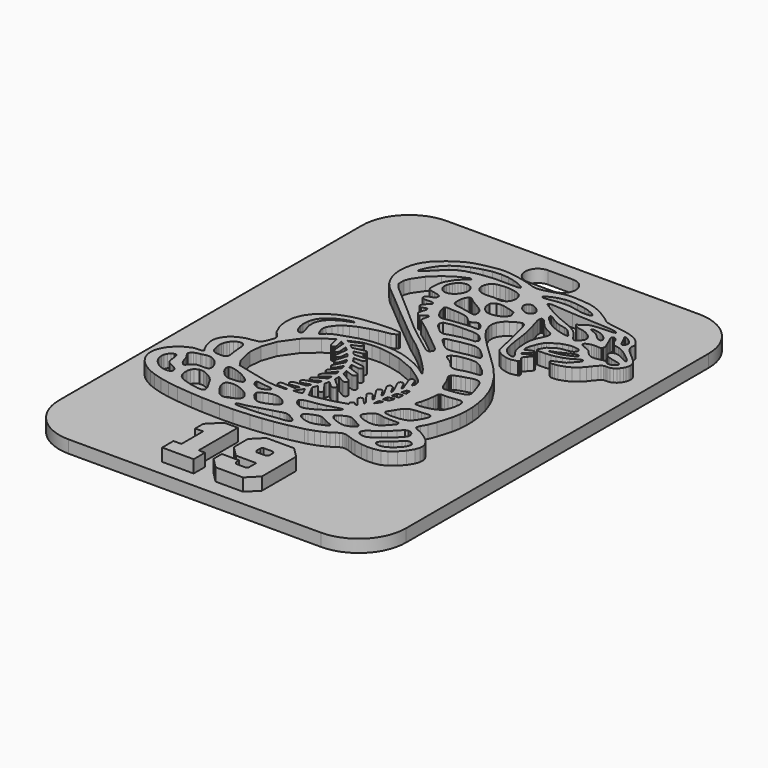
from build123d import *

# Parameters (mm, degrees)
F1_DEPTH = 2.54
F2_W     = 69.85
F2_H     = 95.25
F3_DEPTH = 2.54
F4_R     = 9.525
F6_DEPTH = 2.54


# Not quite as in the source:
# - ends of sketch curves that miss each other by under 0.0002 mm in the source are joined


with BuildPart() as f1:
    # F0 (on Top) → F1 (new body)
    with BuildSketch(Plane.XY):
        Polygon((-8.2281780429, 31.2462601157), (-10.0958576986, 30.7675389293), (-11.1380639944, 30.3636480727), (-12.4204415795, 29.652883082), (-13.8704177588, 28.6461216518), (-15.2257169463, 27.4888991275), (-15.8284643763, 26.846827805), (-16.5017936781, 25.9114281568), (-16.9868772898, 24.9886917871), (-17.2888461994, 24.1974729035), (-17.5726924591, 23.0136513372), (-17.6335459776, 22.5497689682), (-17.6740602593, 21.6151492301), (-17.6280045105, 20.8667022631), (-17.4269723981, 19.7555765356), (-17.20430804, 19.0304242543), (-16.7360745931, 17.9797210423), (-16.2140889153, 17.1404145386), (-15.6879573991, 16.5027353419), (-14.947678965, 15.7886249469), (-14.0724965927, 15.0634110938), (-12.5609690806, 13.8050465328), (-9.0886857893, 10.8515677067), (-5.342140924, 7.7478125022), (-2.8091978797, 5.6307257787), (-1.5091902196, 4.6283359503), (0.1423311709, 3.4050673477), (1.563163338, 2.2145549728), (3.5199169465, 0.3846804372), (5.5455078909, -1.6626453726), (6.1076589433, -2.2972254525), (6.8524115989, -3.2890454455), (7.0789960319, -3.6056479331), (7.0395079477, -3.7197611077), (6.1721041534, -3.0787570307), (5.0096069734, -2.3217515755), (3.8088120985, -1.7146325437), (1.7273139082, -0.8504920577), (0.0306808706, -0.3511648232), (-1.4594196354, -0.0862826953), (-2.7848359484, 0.0338439973), (-4.4325809316, 0.0443522608), (-6.0681552112, -0.0942459888), (-7.6592130383, -0.3793647336), (-9.5361079486, -0.9377804267), (-11.8733961559, -1.7510830829), (-12.6301963716, -2.0678087142), (-13.172562334, -2.4256438218), (-13.62142117, -2.8594996487), (-13.8745841211, -3.0896347254), (-14.0119304096, -3.1911872411), (-14.185008899, -3.1720383937), (-14.4263295297, -2.6863595874), (-14.7089238284, -1.8951612278), (-14.7727943678, -1.2952461032), (-14.6445196662, -0.7206575357), (-14.147203779, 0.1498248515), (-13.4946241929, 0.8740946028), (-12.8925335294, 1.3693170469), (-12.0459410226, 1.8987118715), (-10.7370054432, 2.4979291817), (-8.958543408, 3.0819382433), (-7.4131513747, 3.4864653423), (-6.2016635207, 3.7161283681), (-5.2402600249, 3.9098744774), (-4.4449568748, 4.2413363065), (-4.2034515286, 4.5321812339), (-4.2377060049, 4.9084058028), (-4.4755170398, 5.1506500113), (-5.1994789318, 5.2198157305), (-6.0173789533, 5.3073709108), (-7.4621420487, 5.2495344133), (-9.2230561048, 5.1676848917), (-12.0609850796, 4.8602976587), (-13.9591838523, 4.4160977599), (-15.9473596317, 3.6696210923), (-17.7325124754, 2.6187536887), (-19.0329100906, 1.4390779606), (-19.8561873876, 0.3138112301), (-20.3619796671, -0.7178252303), (-20.6945703135, -1.8480587573), (-20.7833158831, -3.0535330933), (-20.6529682622, -4.2906348398), (-20.3346828106, -5.4881458823), (-19.720175156, -6.8209097702), (-18.8984371554, -7.7585670532), (-18.5574522125, -8.2426244673), (-18.5128126164, -8.5026424185), (-18.66171389, -9.0847427525), (-19.0896998665, -10.1552105305), (-19.3077873832, -10.6363124954), (-19.3952194198, -10.823080461), (-19.5230836424, -10.9713249682), (-20.0220619698, -11.1893303891), (-21.0657459901, -11.3813114385), (-22.2214497419, -11.5752627874), (-23.3337863825, -11.996332192), (-24.0131702503, -12.3898584526), (-24.7578613341, -13.0130887869), (-25.3504699316, -13.7868007393), (-25.6892382876, -14.5173918679), (-25.8122793814, -15.0092073359), (-25.8467801452, -15.595576652), (-25.7631450397, -16.2746937083), (-25.5535954872, -17.0447113492), (-25.4211133753, -17.4274420109), (-25.0605075341, -18.2154181101), (-24.7159924715, -18.7689080546), (-24.6677201357, -18.8595213039), (-24.6881209443, -19.0501888204), (-25.0308504231, -19.1392012013), (-25.7215840364, -19.1855032376), (-26.1809716599, -19.2103782678), (-26.5443892825, -19.2721143162), (-27.3716892742, -19.6063468787), (-28.0206771686, -19.9679994415), (-28.7905100939, -20.5251016016), (-29.4208211918, -21.1146316064), (-29.9690570046, -21.7761596356), (-30.3697256006, -22.415706512), (-30.7029935374, -23.1830765631), (-30.8776934191, -23.8991367335), (-30.9240570272, -24.5455386099), (-30.876441458, -25.1101935845), (-30.7473663222, -25.6701896219), (-30.4887029519, -26.3609437592), (-30.2370587732, -26.8394802301), (-29.6598020919, -27.6332235598), (-29.088415261, -28.206642262), (-28.1307676485, -28.9230923875), (-26.9608202739, -29.5598274824), (-25.6898745302, -30.0719206153), (-24.0739621969, -30.5487535982), (-22.1714328702, -30.9419104277), (-20.1395410725, -31.2260645467), (-17.1374204796, -31.5122300131), (-14.8925105813, -31.6548509573), (-11.3057036364, -31.75), (-8.6367688845, -31.7091162871), (-5.3569386935, -31.5193518245), (-3.1109205019, -31.2946966431), (-0.9777019518, -31.0051652485), (1.5435424396, -30.5608011581), (4.337406489, -29.9279040423), (4.9370958501, -29.7589919152), (5.9386031485, -29.4248824963), (6.9207768839, -29.0279903075), (7.7674309626, -28.6199536126), (8.2726280474, -28.3307916492), (8.9759223196, -27.8459132771), (9.5296995994, -27.5060776756), (9.9716829114, -27.331767749), (10.2292790362, -27.2936137218), (10.7020482765, -27.3414755784), (11.3129642395, -27.5130147714), (12.2242277198, -27.8546359568), (13.03843343, -28.0966133539), (14.6348685326, -28.3984591198), (15.7869805927, -28.5070923992), (16.9305136408, -28.4916173392), (18.3728343859, -28.2090640884), (19.3723098131, -27.7017530364), (20.5650798226, -26.7484154539), (21.4969288271, -25.7102113288), (22.2529696565, -24.485731813), (22.5528861709, -23.6063009826), (22.6021436563, -22.830167204), (22.4525445683, -22.2410271543), (22.1046430535, -21.6120501134), (21.5689678995, -20.9829088808), (20.7981293005, -20.3279895641), (19.6320814768, -19.5857203067), (18.0839597578, -18.8412960343), (17.8310430941, -18.6388682931), (17.7820318961, -18.4662208067), (17.8314125253, -18.1861304302), (17.9895906253, -17.781664903), (18.6505850318, -16.6351148339), (19.2241063538, -15.1447475166), (20.0612988904, -12.3389180031), (20.3419228897, -10.7201733644), (20.434650106, -9.2487907029), (20.4032279351, -7.6929725018), (20.2038172149, -5.9142436552), (19.6753254442, -3.6030824391), (19.0529776398, -1.8339793261), (18.1165928419, 0.1336314532), (16.4870115564, 2.6515509644), (14.4028042044, 5.0404158638), (11.7791042432, 7.596161019), (8.9855275292, 10.2726691093), (6.7964222572, 12.5526954898), (5.7074418742, 14.12870926), (5.1848404778, 15.5236607232), (5.1331816899, 16.344885625), (5.352849551, 17.23264918), (6.032541278, 18.1864793374), (6.7197037236, 18.7081571559), (7.7446698995, 19.31689758), (8.4808435431, 19.6174913848), (8.7462798177, 19.662110457), (9.053954386, 19.5342051865), (9.2906776514, 19.1477391655), (9.5775204082, 18.2618022422), (9.8677290932, 16.9917595524), (10.834263577, 13.1887532943), (11.0390926205, 11.8791609485), (11.4717170102, 10.3329069092), (11.9607001728, 9.7361524732), (12.7906067064, 9.2087895199), (13.9503742007, 8.8610727207), (14.9139942833, 8.7772939476), (16.1735287096, 9.0840038902), (16.347448681, 9.2895102242), (16.3674595345, 9.5117435792), (16.221924189, 9.7619100333), (15.9084618661, 10.1001858145), (15.837572135, 10.2823769387), (15.8998828541, 10.5336722102), (16.0684871219, 10.7846596224), (16.4075633372, 11.1428231133), (17.0936174894, 11.9521441227), (17.0494499441, 12.3008460717), (16.732683265, 12.2797679727), (15.8150984073, 11.7842787172), (15.0990177129, 11.3454971418), (14.8941476215, 11.4280650018), (14.9146510498, 11.670863357), (15.3561417869, 12.0663599171), (15.8215429283, 12.3852200394), (16.3334308216, 12.9318344599), (16.3681368249, 13.2268252258), (15.9950524207, 13.3743308707), (15.3028205589, 13.0950204044), (14.6702313023, 12.792948875), (14.4427848634, 12.7538507459), (14.3894841594, 12.9031214507), (14.3610584855, 13.1483416323), (14.353936674, 13.4823894793), (14.4100491595, 13.7212472357), (14.498835777, 14.1628200686), (14.7819842224, 14.9135246704), (15.0271017842, 15.5714199601), (15.3040314721, 16.0905733326), (15.5397285398, 16.4512612696), (15.7826705627, 16.6768605528), (16.1297305955, 16.8937576803), (17.1537116216, 17.6541085397), (17.995316808, 18.0185113121), (18.999615364, 18.2874777065), (19.7587758341, 18.3525386351), (20.4528958996, 18.2983143533), (21.0168530598, 18.2007024363), (21.3530559218, 17.9078872094), (21.3694956075, 17.615277222), (21.2827203374, 17.2942620847), (20.9964112033, 17.0079324267), (20.484502786, 16.8344024104), (19.7045515523, 16.7040342656), (19.0104520108, 16.6281161662), (18.424801033, 16.4546066738), (17.7849257734, 16.205158558), (16.754602846, 15.4025899288), (16.2994021088, 14.6136697279), (16.0761630801, 14.2962257583), (16.0630893225, 14.0488916096), (16.136790835, 13.9380827914), (16.269231899, 13.8613232099), (16.4453479333, 13.8129893023), (16.8682029217, 13.7790426853), (17.8758674059, 13.8107111436), (18.9218295849, 13.9036846474), (19.8006446967, 14.0631352325), (20.9053669511, 14.3650220463), (21.9472448636, 14.7667784118), (22.7663147504, 15.2334930862), (23.4398082439, 15.6252748109), (23.7038899376, 15.6872776707), (23.9646467511, 15.7318967429), (24.1143484589, 15.5621841816), (24.1351802704, 15.2637248679), (23.8644693401, 14.9652450301), (23.5979863439, 14.656195357), (23.1121022981, 14.0939622088), (22.4531397629, 13.4007246733), (21.5882809386, 13.0305751943), (20.6687257815, 12.6129948616), (20.2689191915, 12.4486390519), (20.1267702982, 12.3242433772), (20.124266376, 12.1040829413), (20.3203522159, 11.9487781946), (20.6240246135, 11.786084825), (20.9493908287, 11.7535543607), (21.3615117901, 11.786084825), (22.0122442205, 11.883696742), (23.1888413556, 12.2794395894), (24.0884061832, 12.7236600122), (25.0990261164, 13.4955042848), (25.8153325743, 14.2562450993), (26.2896821589, 14.8887522601), (26.9574084218, 15.6792117574), (27.3181374067, 16.0484376586), (27.6401171698, 16.2497571063), (27.9280887439, 16.3047612984), (28.3638532983, 16.2896351455), (28.8693582425, 16.3261883045), (29.4282049386, 16.5455688302), (29.9020209005, 16.884029327), (30.2338316366, 17.2422338657), (30.5140656808, 17.6528976265), (30.7363606077, 18.0986573457), (30.8880941868, 18.590760149), (30.9240316272, 18.9710895083), (30.867364995, 19.395114362), (30.6497700532, 19.9153555039), (30.1435057228, 20.5675861828), (29.0852291724, 21.5027395436), (28.2911985073, 22.1658889651), (27.6971532331, 22.7558499728), (27.3140120923, 23.2695439739), (27.0744359976, 23.7597790976), (27.0528447998, 24.0224241147), (27.1311231537, 24.3673291324), (27.1803806391, 24.6259514549), (27.1202044111, 24.8888017115), (26.8265271782, 25.3891346197), (26.2102749876, 26.0746551491), (25.6260606865, 26.5040778023), (24.7185941374, 26.9510689585), (23.6292237993, 27.28835959), (22.4830021134, 27.5173863733), (19.8549921223, 27.9070541309), (19.0187847354, 28.0869055245), (18.4877479946, 28.3549072931), (17.6594833772, 29.0080410259), (16.1305720775, 29.964990824), (14.8880930556, 30.6054202303), (13.9080538112, 30.9904290508), (12.8522401351, 31.2396514031), (11.0529668122, 31.4290464346), (9.4259304968, 31.5157396089), (8.1718759658, 31.4638550576), (6.8842647728, 31.1987061183), (5.5986033554, 30.7903820881), (3.8220910956, 30.3162993149), (3.052812317, 30.2314738202), (2.5093585851, 30.2679448833), (1.9189050025, 30.4165793456), (0.5883577014, 30.8681268193), (-0.7917549444, 31.2065462681), (-2.3376806005, 31.5184282466), (-3.3967370611, 31.6696487269), (-4.5497521751, 31.75), (-5.5576834706, 31.7197682183), align=None)
        Polygon((-26.759582922, -24.733825348), (-26.6166335945, -25.1517956357), (-26.3761133979, -25.4887784079), (-26.0296690838, -25.7474417782), (-25.2160585683, -26.1086017662), (-24.8611583858, -26.2953286838), (-24.5108760926, -26.5698775932), (-24.2769030368, -26.8857412185), (-24.1925085451, -27.1663241698), (-24.2551886953, -27.4858000107), (-24.5195372004, -27.7267922582), (-25.0954803488, -27.8368416902), (-25.7274949347, -27.7817964502), (-26.3844461226, -27.5969166883), (-27.0999726702, -27.2360645596), (-27.962450716, -26.4982284759), (-28.4078204801, -25.8707291595), (-28.6838060661, -25.1937465942), (-28.7662097345, -24.514998969), (-28.7052946442, -23.9864866743), (-28.4672988937, -23.4257722985), (-28.049739085, -22.9743684925), (-27.5664410572, -22.7001069185), (-27.2383451564, -22.6899065142), (-26.9941306484, -22.9745737321), (-26.8677441504, -23.5810154734), align=None, mode=Mode.SUBTRACT)
        Polygon((-22.202916613, -27.5599325263), (-22.3819265246, -26.9413611291), (-22.4322102076, -26.0260749541), (-22.2596858649, -25.3087628226), (-21.9461824942, -24.8590625046), (-21.2046315751, -24.4321642976), (-20.3707023468, -24.4497328008), (-19.4872898697, -24.7880906777), (-18.3880269866, -25.4511990513), (-17.6717410527, -26.1620871857), (-16.7023126917, -27.8573245945), (-16.3128706975, -28.6299282534), (-16.200461011, -29.1731356979), (-16.4079992162, -29.4533697421), (-16.8004582314, -29.536389129), (-17.5492335817, -29.513176539), (-18.9130912573, -29.2795934383), (-20.8303157337, -28.7326711584), (-21.7562743639, -28.1908798667), align=None, mode=Mode.SUBTRACT)
        Polygon((-24.342148681, -20.2197872878), (-24.0994734695, -20.1636748023), (-23.470722192, -19.970359696), (-22.7253332938, -19.9014402643), (-22.2301929456, -20.025835939), (-21.7044103365, -20.2916005968), (-21.1895259462, -20.6784770969), (-20.7276754485, -21.1654283882), (-20.293224427, -21.8756597562), (-20.1027621501, -22.4481754045), (-20.0719556977, -22.8336152279), (-20.1209668957, -23.0471259033), (-20.3133173763, -23.2723762794), (-20.6286268549, -23.3885828971), (-21.0614359601, -23.4046941996), (-22.050731507, -23.3767816245), (-22.5260251934, -23.4221806069), (-22.8593547021, -23.5455706079), (-23.1443092553, -23.7368948909), (-23.427293509, -24.0120389949), (-23.7964783623, -24.4547406451), (-23.9932825405, -24.6317802573), (-24.1245742631, -24.6750037008), (-24.2582262402, -24.6569631467), (-24.457390673, -24.5295299272), (-24.7080702259, -24.2376382781), (-24.8213624424, -24.0560628725), (-25.0115168601, -23.6667029741), (-25.1196575645, -23.3783824928), (-25.2839107545, -22.8382331172), (-25.4733057859, -22.3513228738), (-25.8051165221, -21.8535554596), (-26.0125521076, -21.527511954), (-26.0798501471, -21.2741027154), (-26.0156101765, -21.0225816805), (-25.8401714326, -20.7860020828), (-25.5214960258, -20.5403508982), (-25.0908008876, -20.3568872889), align=None, mode=Mode.SUBTRACT)
        Polygon((-17.1074965572, -23.2132262489), (-17.7370277449, -22.5083926804), (-17.9198961595, -22.2233765554), (-18.1460701134, -21.760951387), (-18.2215366859, -21.5082810107), (-18.2521584226, -21.2161020263), (-18.2186222847, -21.040847998), (-18.1265723588, -20.9170680419), (-17.9316769081, -20.8158233854), (-17.7361657389, -20.7829645378), (-17.4117025776, -20.7937806607), (-16.8161385309, -20.9027012753), (-15.9991005154, -21.1578140019), (-15.2389343715, -21.4770230314), (-14.3613301729, -21.9438813735), (-13.8178969649, -22.3136408974), (-13.5455030705, -22.5398353753), (-13.3366102844, -22.7629102124), (-13.1619104028, -23.0452787476), (-13.1210472139, -23.23857333), (-13.1484672141, -23.353774274), (-13.2810108978, -23.5005000087), (-13.5042088786, -23.6188616414), (-13.9271459628, -23.7302040824), (-14.6808265377, -23.8235675413), (-15.3930487291, -23.8550923319), (-15.9068863979, -23.8169793526), (-16.1946116846, -23.7538887233), (-16.4728138575, -23.6440855787), align=None, mode=Mode.SUBTRACT)
        Polygon((-12.8974592779, -25.1261201715), (-12.3701578965, -25.2927541399), (-11.5050938326, -25.6835301909), (-10.7132387065, -26.2278664527), (-10.1603644805, -26.8242104096), (-9.9091718288, -27.2781386618), (-9.8396572025, -27.5718364186), (-9.8663588644, -27.8504901184), (-10.0593250636, -28.1672978455), (-10.4926267437, -28.5056967704), (-11.726342038, -29.1017533919), (-12.2817407101, -29.2628458932), (-12.7144882435, -29.2847859982), (-13.0222449077, -29.2106329587), (-13.5003708995, -28.9325744535), (-13.9346372054, -28.5016535518), (-14.6941671067, -27.4812847412), (-15.0965391908, -26.7685494511), (-15.2954573361, -26.1941866471), (-15.3317231597, -25.8460593688), (-15.2452762728, -25.4747195006), (-15.0617510917, -25.2422652173), (-14.8546233655, -25.1114455456), (-14.4884760571, -25.0028122663), (-14.0466569368, -24.9644324756), (-13.4231392672, -25.0146751107), align=None, mode=Mode.SUBTRACT)
        Polygon((-4.851166938, -30.08710834), (-6.5055616818, -30.1622875771), (-7.2232637684, -30.1749919035), (-7.8778957497, -30.2128996434), (-8.6038484651, -30.2237157662), (-8.9476862373, -30.2029660505), (-9.198899413, -30.158449598), (-9.3357120787, -30.1119628462), (-9.4727710319, -30.0381792378), (-9.5219669455, -29.8129493857), (-9.3118427222, -29.698446256), (-8.8494380778, -29.6002186205), (-7.6896911074, -29.3679695767), (-5.8136992511, -28.818399707), (-3.5194087237, -28.1618179503), (-2.2662572466, -27.8017457318), (-1.61476543, -27.6151624818), (-1.275155592, -27.5744429605), (-1.0524091381, -27.5818521073), (-0.7409786865, -27.6384161197), (-0.3543074259, -27.7892671689), (0.4216621612, -28.2636167535), (0.8223307572, -28.5158766507), (1.0612295615, -28.7540981646), (1.111739008, -28.9923402024), (0.9787437974, -29.194583228), (0.6180763843, -29.3989196967), (0.0708257212, -29.5412122577), (-0.6144690447, -29.6229591596), (-1.163361624, -29.6759314804), (-3.0051400519, -29.9139682787), align=None, mode=Mode.SUBTRACT)
        Polygon((-5.9171604944, -26.9613719826), (-6.6794611293, -27.1745132268), (-7.1504242618, -27.204108766), (-7.5577426184, -27.1141112353), (-7.9953132806, -26.8809591376), (-8.4064080443, -26.5396252876), (-8.8387040508, -26.0707350742), (-9.1802841883, -25.560550669), (-9.2703843387, -25.2923231369), (-9.2655612099, -25.0973250664), (-9.1131092925, -24.8225914415), (-8.8577913264, -24.6013021882), (-8.4295385385, -24.3461484137), (-7.6373755531, -23.9981237552), (-6.8443095138, -23.7952239632), (-6.3217902132, -23.7631655498), (-5.8916697457, -23.8098985891), (-5.4507126314, -23.9300868535), (-4.9985494392, -24.1331508372), (-4.4363368149, -24.5087186396), (-4.0562126951, -24.8704738221), (-3.8509936964, -25.1563724771), (-3.763500088, -25.4378584823), (-3.7734747287, -25.6164989628), (-3.8925752237, -25.8666859409), (-4.1326438933, -26.0924494157), (-4.5617176393, -26.3645559748), (-5.3110266123, -26.7172806183), align=None, mode=Mode.SUBTRACT)
        Polygon((-10.5022730012, -22.082520671), (-9.9462791345, -22.1563248033), (-9.2089561496, -22.2253879027), (-8.7606514603, -22.2807820498), (-8.3507265618, -22.3887996106), (-8.2321391657, -22.4864730994), (-8.1978025936, -22.644404912), (-8.2847831032, -22.8226554374), (-8.4619663831, -23.0065090018), (-8.8382525238, -23.261354917), (-9.219936464, -23.4272294992), (-9.554415314, -23.509407404), (-9.9007570084, -23.5342413862), (-10.2455388824, -23.5004589608), (-10.6516668497, -23.381727897), (-11.0075727059, -23.1915734793), (-11.2879709417, -22.9428231779), (-11.4925742218, -22.6724611548), (-11.6259388635, -22.3687887571), (-11.6433226511, -22.2036530373), (-11.5733770218, -22.0553469582), (-11.4407922902, -21.9896292631), (-11.2334182766, -21.9775817031), (-10.9516038881, -22.0096811644), align=None, mode=Mode.SUBTRACT)
        with BuildLine():
            Line((-4.2176746275, -20.7893064391), (-5.2175194858, -20.8481486102))
            ThreePointArc((-5.2175194858, -20.8481486102), (-4.6245377337, -20.0558732964), (-4.0970094123, -19.2185906677))
            Line((-4.0970094123, -19.2185906677), (-3.4045772108, -20.5774376799))
            Line((-3.4045772108, -20.5774376799), (-4.2176746275, -20.7893064391))
        make_face(mode=Mode.SUBTRACT)
        Polygon((-21.4224933283, -18.4982586962), (-22.2189458197, -18.4766880224), (-22.8653066482, -18.3592089196), (-23.1687532824, -18.2381791731), (-23.316833598, -18.1247843369), (-23.489234797, -17.9098164609), (-23.7110166251, -17.4077390168), (-23.9041059679, -16.6321799088), (-23.9764528997, -15.9574755022), (-23.9532813576, -15.4659678934), (-23.8623602491, -15.0254007342), (-23.6257190795, -14.4605610441), (-23.3892010536, -14.0834949931), (-22.9616255562, -13.6342667261), (-22.3591038897, -13.2917014389), (-21.8191392297, -13.1782039829), (-21.4304771457, -13.2410278007), (-21.185749539, -13.4034748829), (-21.0409735797, -13.5936087766), (-20.9108517224, -13.9666931808), (-20.8636466322, -14.3503474204), (-20.8267035181, -15.0055745963), (-20.6767760469, -16.3550655053), (-20.5291062104, -17.3481579834), (-20.5083154467, -17.8523699185), (-20.6542407473, -18.2021801609), (-20.9341669322, -18.3922730067), align=None, mode=Mode.SUBTRACT)
        Polygon((-12.825194442, -4.1463719793), (-10.7946777491, -2.9304099037), (-10.2791571162, -4.9154249945), (-10.1506361272, -5.1399775562), (-9.9203573828, -5.2698531261), (-9.6619197759, -5.2637164643), (-9.3606486807, -5.0298665523), (-9.3128894438, -4.6639860553), (-9.7389256448, -3.0235270751), (-8.9664656536, -3.4575470936), (-8.8077744547, -5.873483086), (-8.7207939451, -6.1222333874), (-8.5300032848, -6.2849883288), (-8.2534635521, -6.3299357843), (-7.9269685195, -6.1580271601), (-7.8115007641, -5.8075806753), (-7.9182047919, -4.1829046144), (-7.2518741578, -4.7418744542), (-7.5419596991, -7.0903071676), (-7.5047292497, -7.3473286218), (-7.3546786347, -7.5401511533), (-7.0896528392, -7.6419499565), (-6.7300937195, -7.5348559736), (-6.5509811881, -7.212239968), (-6.3574608423, -5.6455440722), (-5.8134119158, -6.3070310535), (-6.5265782089, -8.5227558917), (-6.5361423707, -8.7908192321), (-6.4230964416, -9.0040220482), (-6.192058311, -9.1475870943), (-5.8123857181, -9.1115675581), (-5.57601136, -8.8282343971), (-5.101805443, -7.354984056), (-4.6920652601, -8.0958782086), (-5.7976084725, -10.1200940482), (-5.8576205089, -10.3721281819), (-5.778049146, -10.6250653696), (-5.5741847282, -10.8025154608), (-5.2063955037, -10.8322957156), (-4.9211125673, -10.5982816119), (-4.184774732, -9.2501042358), (-3.9177375892, -10.0471519218), (-5.3808490979, -11.8257576247), (-5.4845771526, -12.0477857403), (-5.4621034249, -12.3104718053), (-5.2998205344, -12.529831807), (-4.9335706063, -12.6361253558), (-4.6094768762, -12.4597014621), (-3.6285345779, -11.2672393119), (-3.5095982745, -12.0971868934), (-5.2910978547, -13.5792830579), (-5.437577302, -13.7857745416), (-5.4617339938, -14.040107358), (-5.3345675856, -14.2959999948), (-5.0035778075, -14.4591038434), (-4.6521666969, -14.3465299653), (-3.4445578698, -13.3418825022), (-3.4764315677, -14.1813737215), (-5.5314949075, -15.3185648683), (-5.7228397144, -15.5089860974), (-5.7849041461, -15.723687162), (-5.7153484719, -16.0030386762), (-5.413933709, -16.2366833487), (-5.0476632569, -16.1919616567), (-3.6343018085, -15.4098554079), (-3.8170676033, -16.2353492918), (-6.0935433402, -16.9819901511), (-6.3025797939, -17.1165657061), (-6.4267086572, -17.3739155435), (-6.3978109324, -17.6323941982), (-6.1501073526, -17.9058758621), (-5.7819486969, -17.9305867006), (-4.1897210045, -17.4083752593), (-4.5206081629, -18.1959614033), (-6.9573554429, -18.5106346394), (-7.2046280197, -18.6166613768), (-7.3505533203, -18.8136297466), (-7.3780964642, -19.0925092099), (-7.186012795, -19.4075724011), (-6.8289986455, -19.5008127162), (-5.093616386, -19.2767116815), (-5.5667140096, -20.0022539178), (-8.092288955, -19.8503561471), (-8.3520811427, -19.9065917763), (-8.5380486741, -20.0786030202), (-8.6146030161, -20.343074669), (-8.4849737336, -20.6885338335), (-8.1517468447, -20.8470403168), (-6.3199020096, -20.9572128925), (-6.4516657832, -21.2078308736), (-8.4853021168, -21.1906933734), (-10.2838160534, -21.0174712164), (-17.1283078448, -19.354312745), (-18.0210997681, -18.0408618961), (-18.7690336364, -14.7794006424), (-18.512114802, -12.2278834214), (-17.5482894799, -9.4582376357), (-15.4144757352, -6.4205490335), align=None, mode=Mode.SUBTRACT)
        Polygon((-1.2448006666, -20.3984277683), (-2.4459854966, -20.4979894607), (-2.4366060504, -20.3681959866), (-2.4588950625, -20.2485618689), (-2.4894141795, -20.1742446378), (-3.5371824664, -18.1180935285), (-3.3336259079, -17.6339540186), (-3.1512295441, -17.1414407362), (-2.1822321861, -18.3905489947), (-2.0442086071, -18.5123381274), (-1.9060618844, -18.5680606578), (-1.7644466138, -18.5803750292), (-1.6347968074, -18.55508952), (-1.5049622854, -18.4881814356), (-1.3896587216, -18.3783577671), (-1.3163061162, -18.2406625714), (-1.2898712657, -18.0954145612), (-1.3044432718, -17.9610647697), (-1.3359680625, -17.8722986762), (-1.3930246498, -17.7789146934), (-2.8075354396, -15.9555257267), (-2.7211501245, -15.5588593014), (-2.6114085518, -14.9238482184), (-1.4255140662, -15.9692562508), (-1.274724589, -16.0602184072), (-1.1072901864, -16.0922768206), (-0.9605849757, -16.0722454432), (-0.813838717, -16.0008426133), (-0.6820954674, -15.8652819086), (-0.612190886, -15.7072474762), (-0.6002869937, -15.5433431934), (-0.629410482, -15.417161935), (-0.7080172191, -15.2798772183), (-0.7921859474, -15.1965294482), (-2.4960228922, -13.6945455738), (-2.4851657214, -13.2451531151), (-2.4967001826, -12.6443759846), (-1.1359005759, -13.4490585809), (-1.0315568026, -13.4954016651), (-0.9040004393, -13.5172801982), (-0.7710668005, -13.5042474885), (-0.6318323084, -13.4474987605), (-0.51847852, -13.3539300621), (-0.4431966631, -13.2452762589), (-0.4003426508, -13.1341185334), (-0.3854833094, -13.0067058378), (-0.4146273216, -12.8468037257), (-0.4806734, -12.7227364343), (-0.5646574126, -12.6338061492), (-0.6776622938, -12.5600635887), (-2.6136867105, -11.4152375316), (-2.7075632681, -10.8645798925), (-2.8111476552, -10.3837857868), (-1.2727748135, -10.9345049978), (-1.1402516538, -10.9480713303), (-1.0057581946, -10.9246124528), (-0.8735223702, -10.8587100421), (-0.7788659024, -10.7716269127), (-0.7043229077, -10.6503303548), (-0.6613867996, -10.4884374194), (-0.6735985512, -10.3257030019), (-0.7474642554, -10.1622297222), (-0.856815873, -10.0489990776), (-1.045985141, -9.9580163972), (-3.1563810561, -9.1983428282), (-3.5436064634, -8.2221826108), (-1.9821441755, -8.4694141397), (-1.7885827817, -8.4614918942), (-1.6226261037, -8.3864152768), (-1.4838020906, -8.2380681499), (-1.4148826589, -8.038944765), (-1.4293520453, -7.8331100478), (-1.5376364174, -7.6389945073), (-1.6741822718, -7.533398773), (-1.8838139202, -7.4740845509), (-4.1048544619, -7.1224066289), (-4.3447999878, -6.7239546198), (-4.6681548557, -6.2361002745), (-3.0880157712, -6.1863502143), (-2.8867373713, -6.1363333426), (-2.7332387324, -6.0188747638), (-2.636673537, -5.8511735499), (-2.6109365009, -5.6958277552), (-2.6514713066, -5.4849236218), (-2.760043014, -5.3276075277), (-2.9061530302, -5.2293798922), (-3.0631817889, -5.1897891883), (-5.425529742, -5.2609867787), (-5.7769408526, -4.8706417307), (-6.1449147927, -4.4958948863), (-4.6021087773, -4.1509693446), (-4.3963766798, -4.0504430265), (-4.2468391637, -3.8390873661), (-4.2253916336, -3.5797467053), (-4.3143424427, -3.3665233653), (-4.4408520844, -3.2459656697), (-4.6206213822, -3.1731466871), (-4.787111683, -3.1703554296), (-7.0716122851, -3.6799856882), (-7.4899314801, -3.3624185749), (-7.921611768, -3.0632614467), (-6.4707530588, -2.4353311273), (-6.3268185816, -2.3400999888), (-6.2116792094, -2.1726040144), (-6.1743050923, -1.9618025008), (-6.2126233112, -1.7912484575), (-6.3113640455, -1.6345686059), (-6.4377710675, -1.5371619285), (-6.573824347, -1.4880481107), (-6.7223972374, -1.4809673472), (-6.8933207118, -1.5302658805), (-8.897936177, -2.3978543905), (-9.02305019, -2.3225520096), (-9.148164203, -2.2472291048), (-7.6637283078, -1.5891080517), (-6.8884770591, -1.264357555), (-6.7230745278, -1.2322786177), (-5.1786676442, -1.0132059512), (-3.5496199814, -0.9944675828), (-1.4650842462, -1.2725055641), (1.0015048604, -1.871004536), (4.4484821186, -3.2917546072), (6.8419443833, -4.9072975094), (7.8962803348, -5.7547314982), (8.3468426588, -6.3605164731), (8.5925554153, -7.1229197278), (8.309776401, -7.8718387457), (7.715669555, -6.3468680449), (7.6178113506, -6.1906807682), (7.4626913194, -6.0782505577), (7.2786119916, -6.0335904376), (7.0941221847, -6.0607025785), (6.940069399, -6.1425521001), (6.8185470777, -6.2820534036), (6.7628040234, -6.4254542581), (6.7542455353, -6.5815183911), (6.7851546074, -6.7088900388), (7.7987299898, -9.3105677992), (7.7319655731, -9.5174081901), (7.6667199288, -9.7247206318), (6.9317571984, -8.1683893319), (6.8352330509, -8.0654206635), (6.7041260439, -7.99036457), (6.528646252, -7.9577520099), (6.378616161, -7.9808825041), (6.2198018184, -8.0616442562), (6.1067148415, -8.180826847), (6.0556307243, -8.2792391981), (6.0240033139, -8.4242203969), (6.0344500056, -8.5610946345), (6.094031039, -8.716933004), (7.2508636081, -11.1937840867), (7.1977681436, -11.4045445525), (7.1462119755, -11.6156949733), (6.3581332567, -10.1813169978), (6.2822356812, -10.0778762784), (6.1460592579, -9.9776167716), (5.9763672207, -9.9284619059), (5.7778800783, -9.9488627145), (5.6343560802, -10.0193624905), (5.4947932048, -10.1667244677), (5.4344938331, -10.3141274929), (5.4226515126, -10.450775967), (5.4610518273, -10.6168352647), (5.5121564684, -10.7150629003), (6.8273108053, -13.1088125003), (6.750489652, -13.5366548091), (5.8146179529, -12.0852009053), (5.6985755268, -11.9936640782), (5.4952242078, -11.9308813082), (5.2987484128, -11.9546890928), (5.1551423189, -12.0292526114), (5.0353645335, -12.1528478519), (4.9645158503, -12.3138172095), (4.952611958, -12.468793573), (4.9764607905, -12.5849591428), (5.0377453119, -12.7083491438), (6.529939261, -15.0474434589), (6.4812564463, -15.4793905582), (5.5126900912, -14.1601519548), (5.3938564076, -14.0451972982), (5.1988172893, -13.9661595581), (5.0352208658, -13.9657080311), (4.838252496, -14.0446021036), (4.7063245308, -14.1693672094), (4.6411815064, -14.2923262074), (4.612099066, -14.4658767477), (4.6399911171, -14.622659219), (4.7075764919, -14.7506671093), (6.3599804124, -17.001364762), (6.3396616996, -17.43559002), (5.2868855684, -16.1825206387), (5.1672309267, -16.0794493504), (5.0421374377, -16.0249172093), (4.9030671372, -16.0068356073), (4.758291178, -16.0306639159), (4.6063318354, -16.1113230483), (4.4855278524, -16.2402545164), (4.4230939896, -16.3814798319), (4.4080499326, -16.5442142494), (4.4544135408, -16.7190988466), (4.5840428233, -16.8981087582), (5.7485308266, -18.2841733501), (5.6027491937, -18.4045258062), (5.4456383392, -18.4780220792), (5.1938299689, -18.2153154903), (5.0689211954, -18.1209463578), (4.9114819576, -18.0690412826), (4.7057498602, -18.0817250851), (4.5532979428, -18.1543388282), (4.4308109957, -18.2740755656), (4.3602496478, -18.411483426), (4.3366676267, -18.5956038017), (4.3533535999, -18.6956170211), (4.4197280615, -18.8401466929), (4.4934090501, -18.9274761098), (1.8927369634, -19.7408813858), align=None, mode=Mode.SUBTRACT)
        Polygon((-17.0540316615, -1.8612351347), (-16.8031263452, -2.8663546487), (-16.5597327953, -3.6243452536), (-16.4050642911, -4.2352817405), (-16.4564152196, -4.4952996917), (-16.6760830807, -4.6544218936), (-16.9531564362, -4.7069221635), (-17.1929993423, -4.604815501), (-17.5128651383, -4.2498537466), (-17.7648582241, -3.7479199702), (-18.0268669987, -2.9561879878), (-18.1359928529, -2.1552817987), (-18.0421573431, -0.9388476722), (-17.8618954704, -0.2345066785), (-17.7237897957, 0.1177253902), (-17.4474758264, 0.6135840768), (-17.0979118715, 1.0705703978), (-16.5366023011, 1.6195861208), (-15.8049849749, 2.1557948975), (-15.1841148951, 2.5121112327), (-14.1636229408, 2.9682355477), (-13.1464148188, 3.2954489186), (-12.5035225382, 3.4408611204), (-12.2226112037, 3.4370231413), (-12.1773558889, 3.3678574222), (-12.18291788, 3.3162191583), (-12.3322296327, 3.2328713882), (-13.1974578881, 2.898495158), (-14.088279512, 2.538197176), (-15.369015181, 1.7577123195), (-16.060323465, 1.1650011022), (-16.6121304454, 0.4706757972), (-16.9646088015, -0.3378858261), (-17.0803638923, -0.9818658761), align=None, mode=Mode.SUBTRACT)
        Polygon((5.2703843108, -27.2848089462), (4.5581415955, -27.5357142626), (4.0361353937, -27.6633321978), (3.5945830848, -27.7093263748), (3.2653788905, -27.6817832309), (2.7681040512, -27.5898564487), (2.3319290178, -27.469770804), (1.9031220832, -27.3109154135), (1.5132490861, -27.1114020736), (1.1785649966, -26.84036276), (1.0419165224, -26.6395358872), (0.9686665368, -26.3733607503), (1.0338300852, -26.1231122004), (1.1062796367, -26.0339971997), (1.2990816442, -25.8501436353), (1.6739516323, -25.615144382), (2.2348301996, -25.3525198888), (2.9078311182, -25.1063145575), (3.283255253, -25.0019502603), (3.5868660788, -24.9639604246), (3.8771363356, -24.9975786585), (4.177894332, -25.0944517131), (4.8657751159, -25.4306545751), (5.2497987867, -25.6500761487), (5.8460606478, -25.9566629476), (6.2951862951, -26.0946660026), (6.6600200704, -26.2577493272), (6.7841899816, -26.5189781916), (6.5804076596, -26.7299849448), (6.4549447395, -26.8056772807), (6.027389766, -26.9602636892), (5.8494470999, -27.0391372377), align=None, mode=Mode.SUBTRACT)
        Polygon((-1.2464220588, -22.187008112), (0.5867773571, -21.9178364781), (2.113000019, -21.5921418797), (3.4294473649, -21.2116072808), (4.3529841687, -20.958731665), (4.7761470164, -20.9013261705), (4.9178238589, -20.9301623235), (4.9415905956, -21.027938432), (4.7989080795, -21.2616857243), (4.2856450814, -21.7615465816), (3.6608959746, -22.2625362563), (2.8040620156, -22.8715024438), (1.8570458104, -23.4644804725), (1.2890659555, -23.7845925559), (0.7520977926, -24.0503982616), (0.1150548383, -24.3049157936), (-0.2913194164, -24.4121944921), (-0.74374942, -24.4447454804), (-1.1235656806, -24.376133908), (-1.5348656839, -24.1774620501), (-1.9653761065, -23.8357382449), (-2.2963864085, -23.4549984066), (-2.4714351974, -23.1643176707), (-2.5302363206, -22.920862549), (-2.4904814251, -22.7521967093), (-2.3654905558, -22.6016945674), (-2.1511589223, -22.4652718567), (-1.8500725427, -22.3426617659), align=None, mode=Mode.SUBTRACT)
        Polygon((9.5729846148, -24.6816534613), (8.918988876, -24.9391059185), (8.664471344, -25.0152292574), (8.3896145753, -25.0561540182), (8.127934184, -25.0445785091), (7.8379512625, -25.0088873561), (7.51488373, -24.9455299155), (6.9505160907, -24.7958897796), (6.6061036479, -24.677507623), (6.1700312342, -24.495644882), (5.6948196436, -24.2326099098), (5.4629605549, -24.047668576), (5.248813637, -23.7782096068), (5.1769387562, -23.5258470898), (5.2638166461, -23.3471245135), (5.3958677549, -23.2038262788), (5.6585948678, -23.0015216814), (6.0826402455, -22.7389792841), (6.7200115829, -22.4139825), (6.9750627376, -22.3044051189), (7.1893943711, -22.2481900137), (7.48736111, -22.2319966153), (7.7886732531, -22.2880680529), (8.0861884651, -22.3869729788), (8.6550508499, -22.6743493584), (9.1895561386, -22.9963085975), (9.5112485664, -23.180531593), (9.8984124018, -23.3670122232), (10.2017564162, -23.5520561768), (10.3925470764, -23.8416696671), (10.3682672409, -24.0806300433), (10.1827307125, -24.3147467668), (9.9969478966, -24.452195675), align=None, mode=Mode.SUBTRACT)
        Polygon((10.1774150088, -21.7800797105), (9.3915939247, -21.5369940199), (9.040203338, -21.3882979858), (8.5534983341, -21.0677343755), (8.3297872545, -20.7610039089), (8.3358212965, -20.4005622593), (8.4893404594, -20.0807580352), (8.8062713302, -19.7265556671), (9.4256636854, -19.1411509768), (9.6176652588, -18.9790117539), (9.9396244979, -18.8052149262), (10.2704706084, -18.7352487729), (10.6939618393, -18.7763172014), (11.1824113792, -18.8980037144), (11.6619740477, -18.9859283258), (12.5701589352, -19.0375871137), (13.488113224, -19.033584943), (14.083964606, -19.0017933409), (14.5678373045, -19.062811051), (14.7665912582, -19.3138395111), (14.795037456, -19.4858097071), (14.6779688323, -19.7325486612), (14.3785859407, -20.0667401758), (13.5486178352, -20.9694451681), (13.0697324572, -21.4186734352), (12.7192038765, -21.6685525539), (12.4424589042, -21.8064940371), (12.157073348, -21.8974356695), (11.7420790333, -21.9545333047), (11.4089547642, -21.9582481401), (10.957181527, -21.9241168075), align=None, mode=Mode.SUBTRACT)
        Polygon((14.3068957755, -22.9263219203), (15.0430078472, -22.317273637), (16.0479836936, -21.2570267872), (16.9319503175, -20.3625929476), (17.5155489, -20.160801449), (18.0493358504, -20.2894866297), (18.4706925903, -20.6297121863), (18.7460419338, -21.2484272512), (18.7121363647, -21.6692093204), (18.3182201489, -22.2737218103), (16.8940015297, -23.6737221658), (14.4228971536, -25.6100749658), (13.6955693334, -25.9637231872), (13.2560078479, -26.0445670351), (12.6884384721, -26.0028623641), (12.1491716264, -25.7872582456), (11.8726318937, -25.516239456), (11.7768876564, -25.1736331209), (11.9066195586, -24.7772745549), (12.1997836927, -24.4172023364), (12.9264547464, -23.8661547422), align=None, mode=Mode.SUBTRACT)
        Polygon((13.0740630111, -17.9351019701), (12.401698335, -17.9695822099), (11.97221411, -17.9542713415), (11.502338747, -17.9025304579), (11.0732444771, -17.8017373283), (10.7660830076, -17.6393312941), (10.6725758811, -17.4404747206), (10.7285446989, -17.1649406615), (10.9056869308, -16.9092943122), (11.1788402115, -16.5279592792), (11.5003684476, -15.9892465803), (11.9548303225, -15.2436319186), (12.2673690675, -14.8387148644), (12.53627389, -14.5857161049), (12.8304436978, -14.4100310736), (13.1812185658, -14.2785546354), (13.6827829112, -14.1610960566), (14.0086622252, -14.1125158616), (14.5702796548, -14.0552540348), (15.2438141961, -14.0137546033), (15.8709851293, -13.9803416091), (16.4913626343, -13.9259120877), (16.7286195224, -13.924064932), (16.9067469041, -13.9682940491), (17.0725188665, -14.0816273135), (17.1475954839, -14.2028622995), (17.183656068, -14.4094769269), (17.1257374747, -14.7917971096), (16.8585156163, -15.4596054682), (16.2835370937, -16.4264478113), (15.7989871048, -17.0807308854), (15.3028410828, -17.4670737628), (14.7368930993, -17.6887734951), (13.8962525386, -17.8562489455), align=None, mode=Mode.SUBTRACT)
        Polygon((17.69351209, -24.7775618902), (17.9657212689, -24.5528656609), (18.9129632375, -23.5622360571), (19.3184754863, -23.1883717428), (19.6360836475, -23.0092797353), (20.0160640997, -22.9457581031), (20.4167532196, -23.0560948704), (20.7562809619, -23.3462419835), (20.8763871305, -23.6395908332), (20.8462990165, -24.0192223782), (20.5267000319, -24.6853272488), (20.0376142495, -25.3173007868), (19.2181338837, -26.096205299), (18.45101012, -26.617267399), (17.8212326449, -26.9007237036), (17.0884865013, -27.0249962346), (16.6388477552, -26.9712440036), (16.2471891742, -26.7983091819), (16.0927464335, -26.6081752881), (16.0642591877, -26.3684965736), (16.1476274818, -26.1433077694), (16.3667206722, -25.8376035005), (16.6826048214, -25.5260499052), (17.333686159, -25.0415614881), align=None, mode=Mode.SUBTRACT)
        Polygon((7.9249522962, -15.642412311), (7.4436656157, -16.302318948), (7.4926973376, -15.7393058896), (7.5528940896, -15.1774011246), (8.3435383025, -14.9410883383), align=None, mode=Mode.SUBTRACT)
        Polygon((8.7284034553, -14.1262463857), (7.6590850186, -14.3709739924), (7.7422275492, -13.8378232846), (7.8354473403, -13.3063350168), (9.1016520511, -13.0165573349), (8.9333351186, -13.577559046), align=None, mode=Mode.SUBTRACT)
        Polygon((9.2588450015, -12.3048277184), (7.995082641, -12.5081585134), (8.1135058456, -11.9814933745), (8.241883167, -11.4571474421), (9.3808393737, -11.2738890724), (9.3349272925, -11.7911337173), align=None, mode=Mode.SUBTRACT)
        Polygon((9.394877757, -10.5821497854), (8.4543265968, -10.670895355), (8.6075379004, -10.1530349916), (8.7705596532, -9.6381711252), (9.3200269031, -9.5863070978), (9.3714599275, -10.0831714581), align=None, mode=Mode.SUBTRACT)
        Polygon((15.3549719216, -12.2089808613), (14.2952586945, -12.4277251445), (13.4718377298, -12.4984301601), (13.0114854806, -12.4876140372), (12.7406514066, -12.4286076745), (12.6395914657, -12.3505961319), (12.6054601331, -12.2098839152), (12.6569957772, -11.9052879397), (12.9125395068, -11.1216218706), (13.1812390898, -9.8984558877), (13.3664677589, -8.6617440964), (13.3947702891, -8.2677457848), (13.4192553641, -7.8477641497), (13.4961791372, -7.5653956145), (13.6893916238, -7.3878634275), (14.018185339, -7.3114938011), (14.4693018097, -7.3230898341), (15.1753052435, -7.3034894597), (15.9924458788, -7.2252521537), (16.8086013644, -7.1169472576), (17.47255122, -7.0498749817), (17.8021043214, -7.1376148776), (18.0361184251, -7.3330644749), (18.1789240849, -7.6244019773), (18.2585980676, -8.2287297516), (18.1378146086, -9.2130995499), (17.8420028846, -10.258179199), (17.4963795286, -11.0512862862), (17.0524669651, -11.4831923376), (16.2073727069, -11.9247035986), align=None, mode=Mode.SUBTRACT)
        Polygon((15.6682905768, -5.2786373776), (14.8471067229, -5.4144033218), (14.2313471072, -5.4822144601), (13.8316841848, -5.5174540861), (13.5397514879, -5.560923817), (13.0281714538, -5.6093808683), (12.6951703284, -5.4770629481), (12.3601168078, -5.0460599506), (12.0387117154, -4.3420062923), (11.6338562331, -3.2433386038), (11.394013327, -2.817671834), (11.089602067, -2.3305153031), (10.9005969907, -1.9429615126), (10.8396613764, -1.6874588309), (10.9824054644, -1.3666078852), (11.3175821287, -1.094562898), (11.6730980298, -0.9033822827), (12.412883889, -0.6234355739), (13.1766417245, -0.3996629224), (13.9677579883, -0.1789072919), (14.3724698029, -0.0573849705), (14.7738567373, 0.0148798654), (15.2021095251, 0.0112881737), (15.6254981363, -0.1131280249), (15.9644512079, -0.3559469041), (16.2363730514, -0.7009750655), (16.556834042, -1.3737912685), (16.9356651528, -2.55712026), (17.3019766528, -3.6434120053), (17.3676738239, -4.2062403481), (17.2753981346, -4.5584724168), (17.0068832672, -4.8413950987), (16.4652972149, -5.0722485137), align=None, mode=Mode.SUBTRACT)
        Polygon((-8.0762597483, 11.601225587), (-13.8989665764, 16.6467519149), (-14.9900404025, 17.9202015808), (-14.988973157, 19.2808780438), (-14.60330757, 20.3579955823), (-13.1692579777, 22.448832171), (-11.3029123789, 24.2062366311), (-9.1155311189, 25.6496451457), (-7.3410712544, 26.4325313047), (-6.9700187214, 26.3750026665), (-7.0567324197, 26.0703451191), (-7.9054799415, 25.3961127634), (-8.8124949637, 24.496486364), (-9.8291078911, 22.7770922634), (-10.0941336866, 21.6847459523), (-10.1824072053, 20.4967990715), (-10.1536736721, 19.8732814018), (-9.9495834908, 19.4945529107), (-9.1645833648, 19.1743382076), (-8.7370078673, 19.1487243152), (-7.6710553588, 18.874934792), (-7.3219224069, 18.5394092205), (-7.3744432007, 18.0785849204), (-7.636985598, 17.7850308312), (-8.6099440789, 17.4608344813), (-9.0749963132, 17.0235306305), (-9.0716919568, 16.6417645945), (-8.5111417727, 16.3602991132), (-8.0546685505, 16.3224939931), (-7.0314674345, 16.3700890384), (-6.6386800361, 16.2114388874), (-6.5623514577, 15.932600472), (-6.694217851, 15.6631004549), (-7.6173852236, 14.844051092), (-7.7631463326, 14.2818179438), (-7.603490508, 14.031938825), (-7.1315011778, 13.844534617), (-6.4304645405, 14.1638257423), (-6.118110511, 14.1707628381), (-6.0278666929, 13.9278208152), (-6.009785091, 13.6388230435), (-6.2708087158, 13.0948972607), (-6.4096327289, 12.0815065938), (-6.0903416036, 11.6997405579), (-5.6252893693, 11.5262105415), (-5.1671742309, 11.8940818618), (-4.5355496001, 12.407734815), (-4.3358310207, 12.342386551), (-4.2714679064, 12.1701700676), (-4.5355496001, 11.0056410164), (-4.4900069501, 10.4645064911), (-2.1381262126, 8.7386678694), (3.3506969601, 4.2512493754), (3.668428265, 3.5363385463), (3.1918210456, 2.9273518348), (2.4769102166, 3.0332554285), (-1.1505752017, 5.7604987288), (-3.684359728, 7.7387409153), align=None, mode=Mode.SUBTRACT)
        Polygon((-1.1448079712, 17.4765763527), (-2.5832291653, 17.7627212951), (-2.9792388242, 17.8007111307), (-3.3870087077, 17.8589375833), (-3.739384444, 18.0260230786), (-3.95092482, 18.332815117), (-4.0591270963, 18.8563400913), (-4.0350114524, 19.7091513556), (-3.9568972901, 20.1426993231), (-3.8015925433, 20.6369366175), (-3.5408152059, 21.0962216212), (-3.3139639616, 21.2810192873), (-2.981906938, 21.2697721615), (-2.7130021155, 21.1141800794), (-2.1940129347, 20.6813299262), (-1.4419127041, 20.207657632), (-0.3286524856, 19.571394588), (0.4097993168, 19.0327434609), (0.8488682275, 18.4980739806), (1.0055070311, 18.032303408), (1.0596081693, 17.4981470265), (1.0044603095, 17.2394220843), (0.8284879429, 17.107576215), (0.2878665164, 17.1642428472), align=None, mode=Mode.SUBTRACT)
        Polygon((-8.4164032091, 23.2683125368), (-8.1756572491, 23.6024424796), (-7.8358216475, 23.961673216), (-7.4785612105, 24.2352164517), (-7.041996222, 24.4371926659), (-6.5192511579, 24.533470526), (-6.035152696, 24.4594406302), (-5.5686432611, 24.238110329), (-5.1471428535, 23.7911396967), (-4.8687559651, 23.2118511441), (-4.8612852465, 22.5841465882), (-5.0180061459, 22.0025183051), (-5.2854127199, 21.4892758309), (-5.6293736358, 21.0378720249), (-6.0437932799, 20.6571527105), (-6.4822875199, 20.3854566305), (-7.0332119704, 20.229618261), (-7.7404263174, 20.2685521984), (-8.3606601547, 20.6752958843), (-8.7525855471, 21.2242295114), (-8.8547948294, 21.8105577796), (-8.8194320596, 22.2917828883), (-8.6563692589, 22.8112851679), align=None, mode=Mode.SUBTRACT)
        Polygon((-9.458547933, 27.8151478727), (-10.6574751282, 27.2968359823), (-11.4445686974, 26.7876777746), (-12.252145171, 26.1111672602), (-14.3870056372, 23.9737823478), (-15.1091614214, 23.3528506962), (-15.277847785, 23.2675326266), (-15.3588558246, 23.2805448124), (-15.3907910943, 23.3637899627), (-15.3567418575, 23.6016215215), (-15.1589730535, 24.1763742806), (-14.6670754897, 25.2208382111), (-13.8469178334, 26.4590277271), (-12.647210728, 27.67269112), (-11.4751288623, 28.488230887), (-9.6440434135, 29.3629412084), (-7.6351384423, 30.0294360341), (-6.0279898366, 30.3814628633), (-4.3100118887, 30.512713538), (-2.7880992568, 30.3792052285), (-1.7181240536, 30.1457042237), (-0.5505985053, 29.7763757027), (0.3412903641, 29.3865848014), (0.7918526881, 29.0978948889), (0.8923174344, 28.9574700076), (0.8754262217, 28.8402987641), (0.7255192744, 28.7619383144), (0.3909993765, 28.695461233), (-0.9603592122, 28.6789394514), (-4.4603087911, 28.7056411133), (-7.3002901612, 28.3535321883), align=None, mode=Mode.SUBTRACT)
        Polygon((-0.4556957501, 23.6536907884), (-1.4336415513, 23.5838683028), (-1.9689062263, 23.5674901889), (-2.6464224143, 23.6372716266), (-3.1817281372, 23.8105143076), (-3.7034059557, 24.1901869005), (-4.0566436981, 24.6795189703), (-4.2387322025, 25.4798299647), (-4.1028636386, 26.1266012723), (-3.8236968399, 26.6729283575), (-3.2834243206, 27.1788643047), (-2.8323899458, 27.3801221805), (-2.1794204046, 27.5173453254), (-1.2056204417, 27.5908005505), (-0.435951708, 27.5723084695), (0.2018095846, 27.5070423013), (0.8249372991, 27.3957614322), (1.4967478285, 27.2049092001), (2.1935770556, 26.7983707537), (2.5575693489, 26.1698657637), (2.6798305326, 25.7175999516), (2.7015243501, 25.1171717283), (2.5173218786, 24.4979435646), (2.0877760817, 23.8684944728), (1.2662638446, 23.4746808768), (0.4784314131, 23.5001305776), (0.0122298375, 23.6209756085), (-0.1936254036, 23.6531776896), align=None, mode=Mode.SUBTRACT)
        Polygon((8.6074763286, 5.8555656757), (7.0647318851, 5.54245226), (5.9341904988, 5.343410971), (5.3204422304, 5.27761118), (5.0495876324, 5.2800740543), (4.6102519103, 5.4103190553), (4.2491124463, 5.6134651348), (3.8913183866, 5.8734420381), (3.4656926646, 6.2381937177), (2.5788732114, 7.0737648621), (2.3372241975, 7.3798796101), (2.2891981492, 7.542839791), (2.3329757394, 7.6975082952), (2.4644111296, 7.8236074579), (2.8605849801, 7.9879427437), (3.5748595667, 8.1453614575), (4.901856224, 8.4474535108), (6.4490748891, 8.7242805789), (7.092295553, 8.8075257293), (7.62409168, 8.8186086635), (8.1899575677, 8.7407202647), (8.6959345628, 8.5655072842), (9.2400450612, 8.2450873415), (9.6161259624, 7.9403887463), (10.3791449356, 7.2039482913), (10.8086702085, 6.7266022096), (10.911618353, 6.4845427166), (10.8750446701, 6.2745211132), (10.5703255509, 6.0984256028), (10.1341505175, 6.0240673237), (9.3626141041, 5.9721827724), align=None, mode=Mode.SUBTRACT)
        Polygon((12.0116611463, 1.2841015971), (10.6528728869, 0.8729657854), (10.1411491852, 0.7910957399), (9.5706448842, 0.7826603955), (9.0608299101, 1.0162434962), (8.5137434386, 1.7004710166), (7.589693536, 2.4972724152), (6.7437577957, 2.9932542455), (6.3793550233, 3.4617750277), (6.7350966878, 3.9823445529), (7.5299688349, 4.3901349603), (8.6469028409, 4.6218914293), (10.1479015655, 4.8153296793), (11.2468565893, 4.7538809662), (12.2421246062, 4.2846418457), (12.7969280837, 3.7957407789), (13.7233587648, 3.0930417014), (14.5500225139, 1.994784492), (14.4957982321, 1.6694388008), (14.020750833, 1.5512003118), (13.40297987, 1.4788328562), align=None, mode=Mode.SUBTRACT)
        Polygon((-0.3537327552, 9.8701328336), (-1.1467372227, 10.5164526142), (-1.5271897257, 11.3208068273), (-1.2334919689, 11.9805903206), (0.4687646316, 12.3629925991), (2.3133958889, 12.3986837521), (4.5098076879, 12.4224710127), (5.7299361259, 12.1648954119), (6.7058090079, 11.3662673815), (7.0636851635, 10.6634862082), (6.6871732593, 10.1236652159), (5.4929255252, 10.0186646761), (4.1600384935, 9.8510045101), (2.4346924468, 9.4264460336), (1.1073879301, 9.0235813747), (0.2782202588, 9.2849539068), align=None, mode=Mode.SUBTRACT)
        Polygon((2.0802848391, 13.6170471301), (-0.5838678319, 13.2860983999), (-1.5785611782, 13.0972369912), (-2.2479293572, 13.0313345805), (-2.7570259931, 13.1015264972), (-3.2046533919, 13.4140036704), (-3.521851074, 13.8224508443), (-4.0243595212, 14.8074363612), (-4.2784255262, 15.5352157084), (-4.3303100775, 15.953247568), (-4.2230313791, 16.2393514625), (-3.8569661665, 16.3629877509), (-3.3380590815, 16.3244848165), (-2.4480789397, 16.2561195315), (-1.4990924351, 16.2195868965), (-0.2322514818, 16.0505311017), (0.5672796025, 15.762354288), (1.017164636, 15.3332600181), (1.4996211818, 14.8652318108), (1.831000915, 14.7667784118), (2.139681157, 14.8409930231), (2.6575209965, 15.1240593727), (2.9542357743, 15.2644637301), (3.3224765257, 15.3200425929), (3.6651239087, 15.1732552863), (4.1393913976, 14.6843336955), (4.4086451273, 14.2746345605), (4.5184893198, 13.9470517585), (4.489140068, 13.7618025654), (4.2248736587, 13.660496337), (3.8820005123, 13.6458422351), (2.9472371066, 13.6860486576), align=None, mode=Mode.SUBTRACT)
        Polygon((17.8391911032, 14.7930490707), (17.7751768961, 14.8215978883), (19.2213356202, 15.3517726231), (20.3285207489, 15.9133900527), (21.7535192783, 16.5780992946), (22.1379123801, 16.6267000135), (22.41225605, 16.56457401), (22.5302687755, 16.4698559703), (22.5516342098, 16.3309909093), (22.3365021422, 16.0539586017), (21.5138610877, 15.6562659788), (20.1662583823, 15.1081943576), (19.1517388981, 14.9093172602), (18.0049630656, 14.7647875884), align=None, mode=Mode.SUBTRACT)
        Polygon((3.6001655998, 19.0009929068), (2.7881559526, 18.884827337), (2.4394334797, 18.8881932652), (1.8627104212, 18.9998230415), (1.3775036658, 19.3509878647), (0.997831073, 19.7439394547), (0.5710149618, 20.4313481877), (0.4515245117, 21.5360499181), (1.2825598627, 22.3152417657), (2.0165990153, 22.4354095062), (2.6619746941, 22.3681730386), (3.4577088472, 22.1861050581), (4.1438040473, 22.0106252662), (4.4912745591, 21.9404949214), (5.2450577537, 21.6115164906), (5.6418473228, 20.549894536), (5.2276329182, 19.7175046042), (4.5122295143, 19.2909347804), align=None, mode=Mode.SUBTRACT)
        Polygon((11.1906004361, 16.9383767525), (10.9979215723, 17.8678039306), (10.4391980199, 20.0338402803), (9.9196546924, 21.7594326145), (9.8621260542, 22.2440236514), (9.919408405, 22.5591484144), (10.0590123282, 22.7190505264), (10.2351283626, 22.7442949877), (10.4658381099, 22.6503568582), (10.7498485613, 22.4103497605), (11.4733589264, 21.5582568345), (11.9111553521, 21.0808697049), (12.273587825, 20.7625432053), (12.7885748351, 20.4206552086), (13.9719243506, 19.8219920451), (14.3362655511, 19.5208235696), (14.4706974384, 19.2308611721), (14.4409787556, 18.6934825301), (14.044394426, 17.7461995135), (13.7471460255, 17.1211220235), (13.469600619, 16.4041382752), (13.3132901986, 15.7458530304), (13.2377620543, 14.7387016451), (13.2969326087, 13.4925283117), (13.4028156784, 12.4940790822), (13.5382942873, 11.9052263679), (13.8477339155, 11.2871885935), (14.3024215539, 10.6735839927), (14.6409641464, 10.1056246618), (14.6737408982, 9.8826934924), (14.5447889061, 9.7554244644), (14.3135044881, 9.7488567997), (13.8834045445, 9.8510045101), (13.2522724886, 10.1535891383), (12.6719782624, 10.6507203099), (12.3934271823, 11.0268012111), (12.1088010123, 11.6176857967), (11.8583677468, 12.4733498904), (11.600771622, 14.0374802922), (11.4409516058, 15.3317412456), align=None, mode=Mode.SUBTRACT)
        Polygon((11.7925474319, 23.6648763424), (12.7051039213, 23.121607326), (13.5716662336, 22.7918489851), (14.81827057, 22.5327135638), (15.2526394956, 22.41829253), (15.6729495139, 22.1665662555), (16.8158873674, 20.9420046439), (16.9160853024, 20.7610860047), (16.9209905269, 20.7173084146), (16.8780749428, 20.6748443573), (16.6601516177, 20.6345353151), (16.5101830985, 20.6405077852), (15.7279126581, 20.7866998972), (14.5936769604, 21.0697457228), (13.2587785814, 21.5958977629), (12.2548289327, 22.2178556122), (11.121434717, 23.2188292879), (10.6666239349, 23.7473621065), (10.512222242, 24.0685619594), (10.5303448919, 24.2243182331), (10.6331083209, 24.2950027247), (10.8139038163, 24.2787477545), (11.2001440739, 24.0687877229), align=None, mode=Mode.SUBTRACT)
        Polygon((6.1951730757, 22.9488366959), (5.7989376534, 23.1958424614), (5.5090983995, 23.4553678377), (5.2706100743, 23.7480599209), (5.0978599681, 24.0615427677), (5.0195610902, 24.3189131291), (5.0102432159, 24.6370343891), (5.0970800579, 24.9094693314), (5.1831985616, 25.05278809), (5.3766162877, 25.2491817892), (5.4772657496, 25.307326146), (5.7116082365, 25.3720997393), (5.9113473399, 25.3771075836), (6.1238112937, 25.3531356074), (6.4218806524, 25.272928002), (6.7248141877, 25.14652098), (7.0208721991, 24.9806463978), (7.2304422756, 24.8335717559), (7.5451770835, 24.557545122), (7.7017337914, 24.3757234289), (7.9006314127, 24.057540597), (7.9951647368, 23.729957795), (7.9813726409, 23.470288751), (7.8753048556, 23.220060725), (7.7288048844, 23.0469822356), (7.5587844639, 22.9093896597), (7.2433107937, 22.7805813353), (6.971060567, 22.750185362), (6.6179254444, 22.7926699432), align=None, mode=Mode.SUBTRACT)
        Polygon((7.757764181, 27.3800195608), (8.3353081976, 27.453864741), (12.7179724394, 27.1366465349), (19.2793363093, 26.8106851251), (21.3327987809, 26.6562218604), (21.916561555, 26.5057197184), (22.1535721557, 26.3362944925), (22.1597909132, 26.2422126954), (22.0604755083, 26.1567509582), (21.6692684542, 26.0559167807), (20.5759780413, 25.9855606724), (18.5075946564, 25.8823867643), (17.4483124324, 25.7132283498), (16.9419865301, 25.5308935579), (16.5460589671, 25.2182932411), (16.3100950879, 24.9705486133), (16.0651006698, 24.806480139), (15.7110214454, 24.6277986106), (15.5794218635, 24.5329369032), (15.5489437944, 24.4563825613), (15.5909973726, 24.3467641323), (15.8714982281, 24.120323367), (16.2931423034, 23.8983568233), (16.6573808841, 23.7809392924), (17.2096599155, 23.7072172559), (17.6705047395, 23.622042854), (18.4437651649, 23.3128289893), (19.1796925211, 22.8448007819), (19.6028553688, 22.4418129793), (19.8939055358, 21.871883349), (19.8773632303, 21.4164978962), (19.6647761328, 21.028389959), (19.1414974459, 20.4253962416), (18.9502347348, 20.2553347731), (18.7749601825, 20.1763380809), (18.6121231453, 20.1716380958), (18.3279279783, 20.3066241298), (17.9944342781, 20.6729972016), (17.515959379, 21.3805809798), (16.9766514855, 22.0633512996), (16.4029044, 22.5812732349), (15.5615455011, 23.1114274457), (14.2373606252, 23.7255861932), (11.7742400665, 24.7420554528), (10.2086114163, 25.5281228244), (8.1815632713, 26.7290818909), (7.7677798697, 27.0414153964), (7.6350309465, 27.2269929727), align=None, mode=Mode.SUBTRACT)
        Polygon((8.8300996387, 28.7966032697), (7.1177452538, 28.5499258875), (6.4305007123, 28.4502000035), (5.9268018759, 28.4099525331), (5.6249150622, 28.4371878178), (5.4906678904, 28.5004221147), (5.4511182344, 28.5890240166), (5.5320647021, 28.7421942723), (5.9419280288, 29.0726709516), (6.5397702342, 29.3916747416), (7.58021147, 29.7786128135), (8.8674737558, 30.0568355104), (10.0401713401, 30.1241951217), (11.4433734321, 30.019153534), (13.0422303611, 29.7267898341), (14.0425472703, 29.4458579755), (15.1017473986, 29.0079178822), (15.5281735547, 28.6775848706), (15.590833181, 28.5096989411), (15.5080600815, 28.4003062755), (15.1124198538, 28.2654844331), (14.4208037105, 28.2137230255), (13.4482351847, 28.2856800022), (12.2151766569, 28.545000139), (11.0051049556, 28.7932373416), (10.0481551575, 28.860104378), align=None, mode=Mode.SUBTRACT)
        Polygon((19.0467383584, 24.8781497802), (19.3346688846, 24.8442647351), (20.2405550895, 24.6389841646), (20.9166551248, 24.3350449555), (21.5126501745, 23.888156419), (21.9078593993, 23.4265316848), (22.0299974392, 23.102273763), (22.0086320049, 22.8953512763), (21.8871507314, 22.7415242541), (21.7221381553, 22.689126604), (21.4777799796, 22.7229706013), (21.1253426714, 22.9011390309), (20.7545569499, 23.2361925515), (20.1856945651, 23.7704310289), (19.5841785722, 24.1395953582), (19.094169212, 24.3326026052), (18.6520217085, 24.4899802711), (18.4844436383, 24.6209230866), (18.4517695063, 24.6919359614), (18.4513179793, 24.7595418601), (18.5143675607, 24.8332638967), (18.6516728013, 24.876979915), align=None, mode=Mode.SUBTRACT)
        Polygon((25.0205835709, 22.6782489093), (25.5757154316, 22.584228684), (26.3416488061, 22.2969959721), (27.3368757751, 21.6955415511), (28.7101744687, 20.6453924858), (29.3466222283, 20.0293250108), (29.4760052234, 19.8012218054), (29.4901257025, 19.7007775831), (29.4484620795, 19.6404576874), (29.319674279, 19.6231765196), (29.043688693, 19.715411161), (28.5848962642, 19.9526885731), (27.719544865, 20.4072120199), (27.2139373011, 20.5986389226), (26.7223270726, 20.675419028), (26.2567001676, 20.6086135634), (25.9905250308, 20.4909292211), (25.7483629181, 20.2730879918), (25.635768516, 19.996158304), (25.6792792948, 19.7162321191), (25.8917432486, 19.4192915778), (26.2656280869, 19.1688583123), (26.5939497512, 19.0305063501), (27.2071643968, 18.8359598067), (28.0381381759, 18.6382525745), (28.9192314465, 18.4280667794), (29.1737489785, 18.3033221976), (29.2702936499, 18.16987546), (29.2766150272, 18.043057959), (29.1977414786, 17.8584860563), (28.9818500248, 17.607970695), (28.5577430753, 17.311358537), (28.1936892101, 17.1869012905), (27.8398767971, 17.1681423981), (27.5869190855, 17.2327723238), (27.3181784546, 17.4185961875), (27.0310483625, 17.6345697372), (26.7360575966, 17.6910721777), (26.2936227578, 17.6395570576), (25.2478042464, 17.4173442264), (24.7758559642, 17.3745107381), (24.2357681604, 17.4291044511), (23.8150887109, 17.5757686139), (23.5193796068, 17.7684885257), (23.1449200978, 18.163841418), (22.8621821315, 18.5093211064), (22.6495950339, 18.7135960033), (22.2200492371, 18.9891505863), (21.2048524625, 19.407592925), (20.7991349742, 19.6097333308), (20.5641357208, 19.8202680331), (20.5022765287, 19.9956862531), (20.5323851667, 20.1317805805), (20.6301202273, 20.2609172881), (20.7874773693, 20.3804693101), (21.1154090785, 20.5364102993), (21.6755693076, 20.6871176808), (22.1434333233, 20.7444205555), (22.612590348, 20.7435995974), (23.1162891844, 20.7083804953), (23.4169445611, 20.7280424416), (23.6091103261, 20.8044325919), (23.775949534, 20.9869315754), (23.8419545645, 21.259674377), (23.8171000583, 21.5295643492), (23.7229156413, 21.8357201451), (23.4677618668, 22.4026943263), (23.2345892452, 22.9149311268), (23.0148392884, 23.5202850987), (22.7307262172, 24.0387406568), (22.6183986265, 24.3756002852), (22.6326832973, 24.544204553), (22.741131861, 24.7456676684), (22.8319913977, 24.8001177138), (23.0249781208, 24.8036273096), (23.2922615511, 24.6683128923), (23.4595933338, 24.5213203463), (23.5949898469, 24.3483034287), (23.7769757316, 23.95650118), (24.023140015, 23.3991732564), (24.3421848529, 22.9796021004), (24.6537384482, 22.7735005718), align=None, mode=Mode.SUBTRACT)
        Polygon((24.8681111296, 25.7763805509), (25.2946193815, 25.5035761775), (25.6593505371, 25.1909553366), (25.9455365274, 24.8240281181), (26.0564479654, 24.5014531605), (26.0368886389, 24.2491727393), (25.9234732787, 23.9837775126), (25.7679838164, 23.7812266277), (25.5713027819, 23.6614488424), (25.4320888137, 23.6682833185), (25.2592566117, 23.7902982146), (24.9927736156, 24.2019266012), (24.5328523694, 25.2141884506), (24.1876600163, 25.7417771674), (24.1201567373, 25.9191451628), (24.1522151508, 26.0341613913), (24.3190748827, 26.0246177535), align=None, mode=Mode.SUBTRACT)
    extrude(amount=F1_DEPTH)

    # F2 (on Top) → F3 (join)
    with BuildSketch(Plane.XY):
        with Locations((0, -4.445)):
            Rectangle(F2_W, F2_H)
        with BuildLine():
            ThreePointArc((-2.54, 34.925), (-5.08, 37.465), (-2.54, 40.005))
            Line((-2.54, 40.005), (2.54, 40.005))
            ThreePointArc((2.54, 40.005), (5.08, 37.465), (2.54, 34.925))
            Line((2.54, 34.925), (-2.54, 34.925))
        make_face(mode=Mode.SUBTRACT)
    extrude(amount=-F3_DEPTH)

    # F4
    f4_edges = [f1.edges().sort_by_distance(p)[0] for p in [
        (34.925, 43.18, -1.27),
        (-34.925, 43.18, -1.27),
        (-34.925, -52.07, -1.27),
        (34.925, -52.07, -1.27),
    ]]
    fillet(f4_edges, radius=F4_R)

    # F5 (on face) → F6 (join)
    with BuildSketch(Plane.XY):
        Polygon((7.1986729821, -36.0721161083), (1.6185977821, -36.0721161083), (-0.4438822179, -38.1442227083), (-0.4438822179, -41.6991559083), (1.5942391821, -43.7379377083), (5.7029431821, -43.7379377083), (5.7029431821, -45.5685157083), (5.3267945821, -45.9530209083), (3.4377203821, -45.9530209083), (3.0365019821, -45.5350639083), (3.0365019821, -44.7075573083), (-0.4491146179, -44.7075573083), (-0.4491146179, -46.7888841083), (1.5904291821, -48.8584761083), (7.1349189821, -48.8584761083), (9.2394105821, -46.7539845083), (9.2394105821, -38.1128283083), align=None)
        Polygon((-0.0908984179, -38.2899679083), (1.7652827821, -36.4250745083), (7.0524705821, -36.4250745083), (8.8864267821, -38.2590307083), (8.8864267821, -46.6077821083), (6.9887165821, -48.5054923083), (1.7381555821, -48.5054923083), (-0.0961308179, -46.6442057083), (-0.0961308179, -45.0605411083), (2.6835181821, -45.0605411083), (2.6835181821, -45.6770753083), (3.2872761821, -46.3059793083), (5.4752829821, -46.3059793083), (6.0559269821, -45.7124575083), (6.0559269821, -43.3849539083), (1.7404923821, -43.3849539083), (-0.0908984179, -41.5529789083), align=None, mode=Mode.SUBTRACT)
        Polygon((7.0524705821, -36.4250745083), (1.7652827821, -36.4250745083), (-0.0908984179, -38.2899679083), (-0.0908984179, -41.5529789083), (1.7404923821, -43.3849539083), (6.0559269821, -43.3849539083), (6.0559269821, -45.7124575083), (5.4752829821, -46.3059793083), (3.2872761821, -46.3059793083), (2.6835181821, -45.6770753083), (2.6835181821, -45.0605411083), (-0.0961308179, -45.0605411083), (-0.0961308179, -46.6442057083), (1.7381555821, -48.5054923083), (6.9887165821, -48.5054923083), (8.8864267821, -46.6077821083), (8.8864267821, -38.2590307083), align=None)
        Polygon((0.2620599821, -38.4356877083), (1.9119677821, -36.7780583083), (6.9062681821, -36.7780583083), (8.5334429821, -38.4052331083), (8.5334429821, -46.4615797083), (6.8424887821, -48.1525339083), (1.8858565821, -48.1525339083), (0.2568275821, -46.4995019083), (0.2568275821, -45.4134995083), (2.3305343821, -45.4134995083), (2.3305343821, -45.8190867083), (3.1368319821, -46.6589631083), (5.6237713821, -46.6589631083), (6.4088853821, -45.8563993083), (6.4088853821, -43.0319955083), (1.8867201821, -43.0319955083), (0.2620599821, -41.4068019083), align=None, mode=Mode.SUBTRACT)
        Polygon((6.9062681821, -36.7780583083), (1.9119677821, -36.7780583083), (0.2620599821, -38.4356877083), (0.2620599821, -41.4068019083), (1.8867201821, -43.0319955083), (6.4088853821, -43.0319955083), (6.4088853821, -45.8563993083), (5.6237713821, -46.6589631083), (3.1368319821, -46.6589631083), (2.3305343821, -45.8190867083), (2.3305343821, -45.4134995083), (0.2568275821, -45.4134995083), (0.2568275821, -46.4995019083), (1.8858565821, -48.1525339083), (6.8424887821, -48.1525339083), (8.5334429821, -46.4615797083), (8.5334429821, -38.4052331083), align=None)
        Polygon((2.3511591821, -39.0517647083), (3.1334029821, -38.2909585083), (5.6163799821, -38.2909585083), (6.4151845821, -39.0517393083), (6.4151845821, -40.7752563083), (5.6169641821, -41.5737053083), (3.1313709821, -41.5737053083), (2.3511591821, -40.7935443083), align=None, mode=Mode.SUBTRACT)
        Polygon((-4.0734152179, -46.0097645083), (-4.0734152179, -36.1585269083), (-6.7948982179, -36.1585015083), (-9.1534914179, -38.5171201083), (-9.1534914179, -40.5318481083), (-7.5568220179, -40.5318481083), (-7.5568220179, -46.0098661083), (-9.1534914179, -46.0098661083), (-9.1534914179, -48.8584761083), (-2.8033136179, -48.8584761083), (-2.8036946179, -46.0097645083), align=None)
        Polygon((-6.6665266179, -36.4684323083), (-4.3637372179, -36.4684323083), (-4.3634324179, -46.3196953083), (-3.0939404179, -46.3196953083), (-3.0938134179, -48.5485707083), (-8.8435860179, -48.5485707083), (-8.8435860179, -46.3197715083), (-7.2469166179, -46.3197715083), (-7.2469166179, -40.2219427083), (-8.8435860179, -40.2219427083), (-8.8435860179, -38.6454917083), align=None, mode=Mode.SUBTRACT)
        Polygon((-4.3634324179, -46.3196953083), (-4.3637372179, -36.4684323083), (-6.6665266179, -36.4684323083), (-8.8435860179, -38.6454917083), (-8.8435860179, -40.2219427083), (-7.2469166179, -40.2219427083), (-7.2469166179, -46.3197715083), (-8.8435860179, -46.3197715083), (-8.8435860179, -48.5485707083), (-3.0938134179, -48.5485707083), (-3.0939404179, -46.3196953083), align=None)
        Polygon((-6.5024934179, -36.8644183083), (-4.7597232179, -36.8644437083), (-4.7594184179, -46.7156813083), (-3.4899264179, -46.7156813083), (-3.4898502179, -48.1525593083), (-8.4475746179, -48.1525593083), (-8.4475746179, -46.7157829083), (-6.8509052179, -46.7157829083), (-6.8509052179, -39.8259313083), (-8.4475746179, -39.8259313083), (-8.4475746179, -38.8094995083), align=None, mode=Mode.SUBTRACT)
        Polygon((-4.7594184179, -46.7156813083), (-4.7597232179, -36.8644437083), (-6.5024934179, -36.8644183083), (-8.4475746179, -38.8094995083), (-8.4475746179, -39.8259313083), (-6.8509052179, -39.8259313083), (-6.8509052179, -46.7157829083), (-8.4475746179, -46.7157829083), (-8.4475746179, -48.1525593083), (-3.4898502179, -48.1525593083), (-3.4899264179, -46.7156813083), align=None)
        Polygon((5.6163799821, -38.2909585083), (3.1334029821, -38.2909585083), (2.3511591821, -39.0517647083), (2.3511591821, -40.7935443083), (3.1313709821, -41.5737053083), (5.6169641821, -41.5737053083), (6.4151845821, -40.7752563083), (6.4151845821, -39.0517393083), align=None)
        Polygon((2.7252757821, -39.2097781083), (3.2853457821, -38.6650751083), (5.4667485821, -38.6650751083), (6.0410679821, -39.2120895083), (6.0410679821, -40.6203163083), (5.4619733821, -41.1995887083), (3.2863109821, -41.1995887083), (2.7252757821, -40.6385789083), align=None, mode=Mode.SUBTRACT)
        Polygon((5.4667485821, -38.6650751083), (3.2853457821, -38.6650751083), (2.7252757821, -39.2097781083), (2.7252757821, -40.6385789083), (3.2863109821, -41.1995887083), (5.4619733821, -41.1995887083), (6.0410679821, -40.6203163083), (6.0410679821, -39.2120895083), align=None)
        Polygon((3.0993923821, -39.3677915083), (3.4372631821, -39.0391917083), (5.3170917821, -39.0391917083), (5.6669513821, -39.3724143083), (5.6669513821, -40.4653763083), (5.3069825821, -40.8254721083), (3.4412763821, -40.8254721083), (3.0993923821, -40.4836135083), align=None, mode=Mode.SUBTRACT)
    extrude(amount=F6_DEPTH)


solid = f1.part
